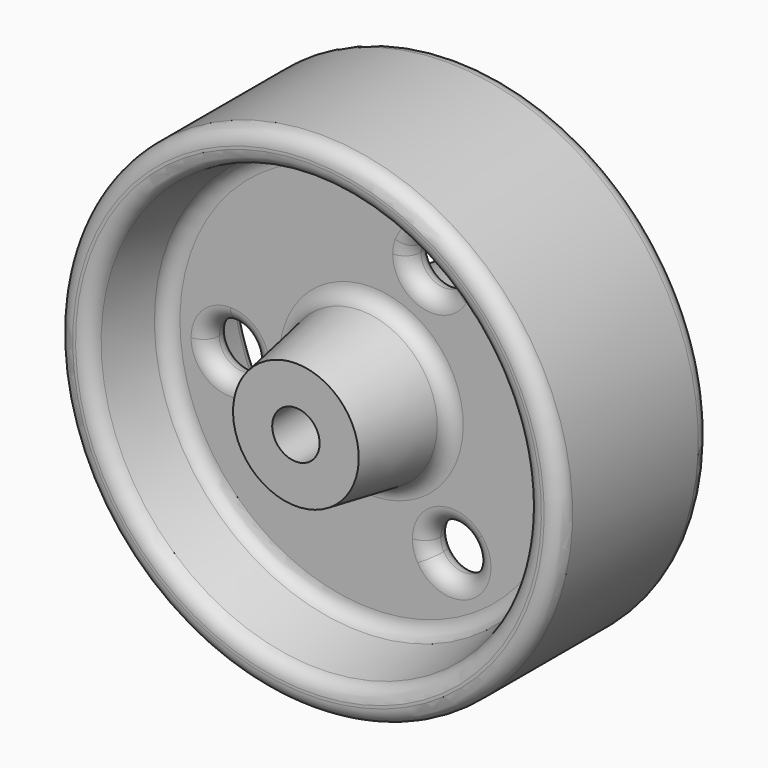
from build123d import *

# Parameters (mm, degrees)
F3_DEPTH = 6.35
F4_R     = 3.17499


# Not quite as in the source:
# - a fillet or chamfer is up to 0.001 mm smaller than in the source, because OpenCascade refuses the exact size


with BuildPart() as f1:
    # F0 (on Right) → F1 (revolve)
    with BuildSketch(Plane.YZ):
        Polygon((15.967091351, 50.8), (15.967091351, 4.7879), (38.192091351, 4.7879), (38.192091351, 12.7), (19.142091351, 15.875), (19.142091351, 41.275), (35.017091351, 44.45), (35.017091351, 50.8), align=None)
        Polygon((-6.257908649, 12.7), (-6.257908649, 4.7879), (15.967091351, 4.7879), (15.967091351, 50.8), (-3.082908649, 50.8), (-3.082908649, 44.45), (12.792091351, 41.275), (12.792091351, 15.875), align=None)
    revolve(axis=Axis((0, 6.442091351, 0), (0, 1, 0)))

    # F2 (on face) → F3 (cut)
    with BuildSketch(Plane(origin=(0, 19.142091351, 0), x_dir=(-1, 0, 0), z_dir=(0, 1, 0))):
        with BuildLine():
            ThreePointArc((-7.4930797023, 25.813395576), (-7.5699539763, 26.6656383857), (-7.7980950541, 27.4903681046))
            ThreePointArc((-7.7980950541, 27.4903681046), (-12.2555797023, 25.813395576), (-16.3726315809, 23.4193842813))
            ThreePointArc((-16.3726315809, 23.4193842813), (-11.0158324139, 21.2150879622), (-7.4930797023, 25.813395576))
        make_face()
        with BuildLine():
            ThreePointArc((-16.3726315809, 23.4193842813), (-12.2555797023, 25.813395576), (-7.7980950541, 27.4903681046))
            ThreePointArc((-7.7980950541, 27.4903681046), (-14.2981763193, 30.115628172), (-16.3726315809, 23.4193842813))
        make_face()
        with BuildLine():
            ThreePointArc((27.706404665, -6.9918356343), (28.3570197509, -3.5227909175), (28.575, 0))
            ThreePointArc((28.575, 0), (28.5482618701, 1.2358677908), (28.4680975191, 2.4694227352))
            ThreePointArc((28.4680975191, 2.4694227352), (23.7357051482, -1.9108786898), (27.706404665, -6.9918356343))
        make_face()
        with BuildLine():
            ThreePointArc((28.4680975191, 2.4694227352), (28.5482618701, 1.2358677908), (28.575, 0))
            ThreePointArc((28.575, 0), (28.3570197509, -3.5227909175), (27.706404665, -6.9918356343))
            ThreePointArc((27.706404665, -6.9918356343), (31.5637229642, -5.9248039342), (33.2453461779, -2.2930544277))
            ThreePointArc((33.2453461779, -2.2930544277), (31.8452237416, 1.0797520252), (28.4680975191, 2.4694227352))
        make_face()
        with BuildLine():
            ThreePointArc((-19.9083096109, -20.4985324703), (-18.9318108882, -27.4403980063), (-12.0954659382, -25.8888070165))
            ThreePointArc((-12.0954659382, -25.8888070165), (-16.2272664756, -23.5203411482), (-19.9083096109, -20.4985324703))
        make_face()
        with BuildLine():
            ThreePointArc((-19.9083096109, -20.4985324703), (-16.2272664756, -23.5203411482), (-12.0954659382, -25.8888070165))
            ThreePointArc((-12.0954659382, -25.8888070165), (-11.6251416235, -24.7458423091), (-11.4647664756, -23.5203411482))
            ThreePointArc((-11.4647664756, -23.5203411482), (-14.622517536, -19.0363488321), (-19.9083096109, -20.4985324703))
        make_face()
    extrude(amount=-F3_DEPTH, mode=Mode.SUBTRACT)

    # F4 (radius 3.175 in the source; OpenCascade refuses exactly that, so slightly less here)
    f4_edges = [f1.edges().sort_by_distance(p)[0] for p in [
        (0, 12.792091, -41.275),
        (-29.259288, 12.792091, 2.405727),
        (0, 12.792091, -15.875),
        (20.359067, 12.792091, -21.151875),
        (17.01808, 12.792091, 25.813396),
        (0, 19.142091, -41.275),
        (-29.259288, 19.142091, 2.405727),
        (17.01808, 19.142091, 25.813396),
        (0, 19.142091, -15.875),
        (20.359067, 19.142091, -21.151875),
        (0, 35.017091, -44.45),
        (0, 35.017091, -50.8),
        (0, -3.082909, -50.8),
        (0, -3.082909, -44.45),
    ]]
    fillet(f4_edges, radius=F4_R)


solid = f1.part
